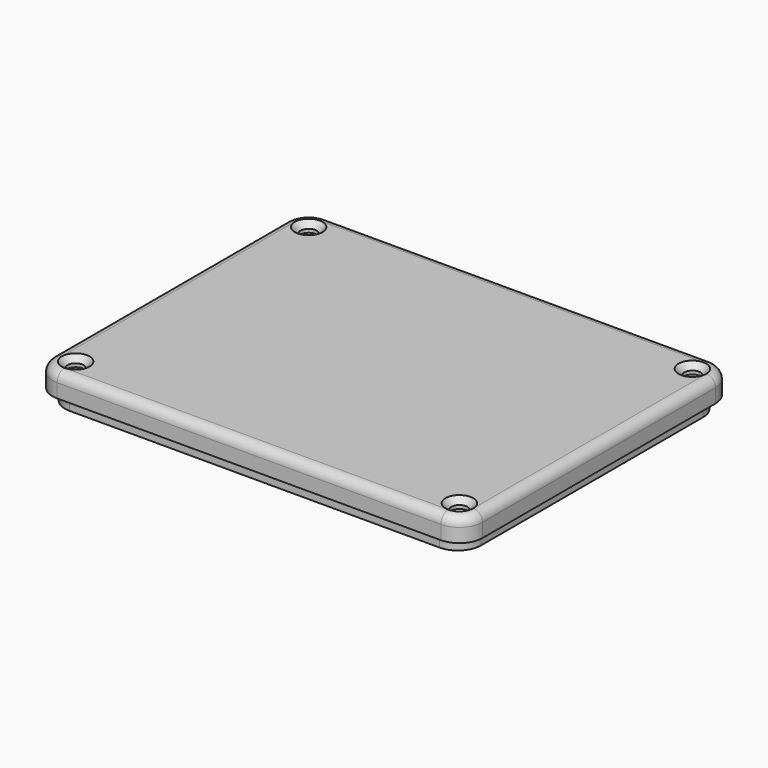
from build123d import *

# Parameters (mm, degrees)
F0_W           = 93
F0_H           = 73
F0_W_2         = 90
F0_H_2         = 70
F0_W_3         = 87
F0_H_3         = 67
F1_DEPTH       = 5
F2_DEPTH       = 3
F3_DEPTH       = 2.5
F4_R           = 2
F5_T1_DEPTH    = 2.5
F5_T3_DEPTH    = 5
F5_T6_ANGLE    = 90
F5_T8_ANGLE    = 90
F5_T10_ANGLE   = 90
F5_T12_ANGLE   = 90
F7_D           = 3.5
F7_DEPTH       = 6
F7_CSINK_D     = 6
F7_CSINK_ANGLE = 90
F7_TIP         = 1.0515060833


# Not quite as in the source:
# - a fillet or chamfer that OpenCascade refuses, or shapes differently, is made with other operations: its cross-section is extruded or revolved along the edge and cut away or added
# - a feature names something its author has since deleted; it is built from what else it names


with BuildPart() as f1:
    # F0 (on Top) → F1 (new body)
    with BuildSketch(Plane.XY):
        Rectangle(F0_W, F0_H)
        Rectangle(F0_W_2, F0_H_2, mode=Mode.SUBTRACT)
        Rectangle(F0_W_2, F0_H_2)
        Rectangle(F0_W_3, F0_H_3, mode=Mode.SUBTRACT)
        Rectangle(F0_W_3, F0_H_3)
    extrude(amount=F1_DEPTH)

    # F0 (on Top) → F2 (cut)
    with BuildSketch(Plane.XY):
        Rectangle(F0_W_3, F0_H_3)
    extrude(amount=F2_DEPTH, mode=Mode.SUBTRACT)

    # F0 (on Top) → F3 (join)
    with BuildSketch(Plane.XY):
        Rectangle(F0_W_2, F0_H_2)
        Rectangle(F0_W_3, F0_H_3, mode=Mode.SUBTRACT)
    extrude(amount=-F3_DEPTH)

    # F4
    f4_edges = [f1.edges().sort_by_distance(p)[0] for p in [
        (-43.5, -33.5, 0.25),
        (-43.5, 33.5, 0.25),
        (43.5, 33.5, 0.25),
        (43.5, -33.5, 0.25),
        (0, -36.5, 5),
        (46.5, 0, 5),
        (-46.5, 0, 5),
        (0, 36.5, 5),
    ]]
    fillet(f4_edges, radius=F4_R)

    # F5: fillet of radius 5 on 8 edges, made by hand

    # F5_s2 → F5_t1 (cut)
    with BuildSketch(Plane.XY.offset(-2.5)):
        with BuildLine():
            ThreePointArc((-40, -35), (-43.5355339059, -33.5355339059), (-45, -30))
            Line((-45, -30), (-45.1, -30))
            Line((-45.1, -30), (-45.1, -35.1))
            Line((-45.1, -35.1), (-40, -35.1))
            Line((-40, -35.1), (-40, -35))
        make_face()
        with BuildLine():
            ThreePointArc((40, -35), (43.5355339059, -33.5355339059), (45, -30))
            Line((45, -30), (45.1, -30))
            Line((45.1, -30), (45.1, -35.1))
            Line((45.1, -35.1), (40, -35.1))
            Line((40, -35.1), (40, -35))
        make_face()
        with BuildLine():
            ThreePointArc((45, 30), (43.5355339059, 33.5355339059), (40, 35))
            Line((40, 35), (40, 35.1))
            Line((40, 35.1), (45.1, 35.1))
            Line((45.1, 35.1), (45.1, 30))
            Line((45.1, 30), (45, 30))
        make_face()
        with BuildLine():
            ThreePointArc((-40, 35), (-43.5355339059, 33.5355339059), (-45, 30))
            Line((-45, 30), (-45.1, 30))
            Line((-45.1, 30), (-45.1, 35.1))
            Line((-45.1, 35.1), (-40, 35.1))
            Line((-40, 35.1), (-40, 35))
        make_face()
    extrude(amount=F5_T1_DEPTH, mode=Mode.SUBTRACT)

    # F5_s4 → F5_t3 (cut)
    with BuildSketch(Plane.XY):
        with BuildLine():
            ThreePointArc((-46.5, -31.5), (-45.0355339059, -35.0355339059), (-41.5, -36.5))
            Line((-41.5, -36.5), (-41.5, -36.6))
            Line((-41.5, -36.6), (-46.6, -36.6))
            Line((-46.6, -36.6), (-46.6, -31.5))
            Line((-46.6, -31.5), (-46.5, -31.5))
        make_face()
        with BuildLine():
            ThreePointArc((46.5, -31.5), (45.0355339059, -35.0355339059), (41.5, -36.5))
            Line((41.5, -36.5), (41.5, -36.6))
            Line((41.5, -36.6), (46.6, -36.6))
            Line((46.6, -36.6), (46.6, -31.5))
            Line((46.6, -31.5), (46.5, -31.5))
        make_face()
        with BuildLine():
            ThreePointArc((41.5, 36.5), (45.0355339059, 35.0355339059), (46.5, 31.5))
            Line((46.5, 31.5), (46.6, 31.5))
            Line((46.6, 31.5), (46.6, 36.6))
            Line((46.6, 36.6), (41.5, 36.6))
            Line((41.5, 36.6), (41.5, 36.5))
        make_face()
        with BuildLine():
            ThreePointArc((-41.5, 36.5), (-45.0355339059, 35.0355339059), (-46.5, 31.5))
            Line((-46.5, 31.5), (-46.6, 31.5))
            Line((-46.6, 31.5), (-46.6, 36.6))
            Line((-46.6, 36.6), (-41.5, 36.6))
            Line((-41.5, 36.6), (-41.5, 36.5))
        make_face()
    extrude(amount=F5_T3_DEPTH, mode=Mode.SUBTRACT)

    # F5_s5 → F5_t6 (revolve, cut)
    with BuildSketch(Plane.YZ.offset(-41.5)):
        with BuildLine():
            ThreePointArc((34.5, 5), (35.9142135624, 4.4142135624), (36.5, 3))
            Line((36.5, 3), (36.5, 5))
            Line((36.5, 5), (34.5, 5))
        make_face()
    revolve(axis=Axis((-41.5, 31.5, 5), (0, 0, 1)), revolution_arc=F5_T6_ANGLE, mode=Mode.SUBTRACT)

    # F5_s7 → F5_t8 (revolve, cut)
    with BuildSketch(Plane.XZ.offset(-31.5)):
        with BuildLine():
            ThreePointArc((44.5, 5), (45.9142135624, 4.4142135624), (46.5, 3))
            Line((46.5, 3), (46.5, 5))
            Line((46.5, 5), (44.5, 5))
        make_face()
    revolve(axis=Axis((41.5, 31.5, 5), (0, 0, 1)), revolution_arc=F5_T8_ANGLE, mode=Mode.SUBTRACT)

    # F5_s9 → F5_t10 (revolve, cut)
    with BuildSketch(Plane.YZ.offset(41.5)):
        with BuildLine():
            ThreePointArc((-34.5, 5), (-35.9142135624, 4.4142135624), (-36.5, 3))
            Line((-36.5, 3), (-36.5, 5))
            Line((-36.5, 5), (-34.5, 5))
        make_face()
    revolve(axis=Axis((41.5, -31.5, 5), (0, 0, 1)), revolution_arc=F5_T10_ANGLE, mode=Mode.SUBTRACT)

    # F5_s11 → F5_t12 (revolve, cut)
    with BuildSketch(Plane.XZ.offset(31.5)):
        with BuildLine():
            ThreePointArc((-44.5, 5), (-45.9142135624, 4.4142135624), (-46.5, 3))
            Line((-46.5, 3), (-46.5, 5))
            Line((-46.5, 5), (-44.5, 5))
        make_face()
    revolve(axis=Axis((-41.5, -31.5, 5), (0, 0, 1)), revolution_arc=F5_T12_ANGLE, mode=Mode.SUBTRACT)

    # F7
    with Locations(Plane.XY.offset(5)):
        with Locations((41.5, -31.5), (-41.5, -31.5), (-41.5, 31.5), (41.5, 31.5)):
            CounterSinkHole(F7_D / 2, F7_CSINK_D / 2, depth=F7_DEPTH, counter_sink_angle=F7_CSINK_ANGLE)
            with Locations((0, 0, -(F7_DEPTH + F7_TIP / 2))):  # 118° drill point
                Cone(0, F7_D / 2, F7_TIP, mode=Mode.SUBTRACT)


solid = f1.part
